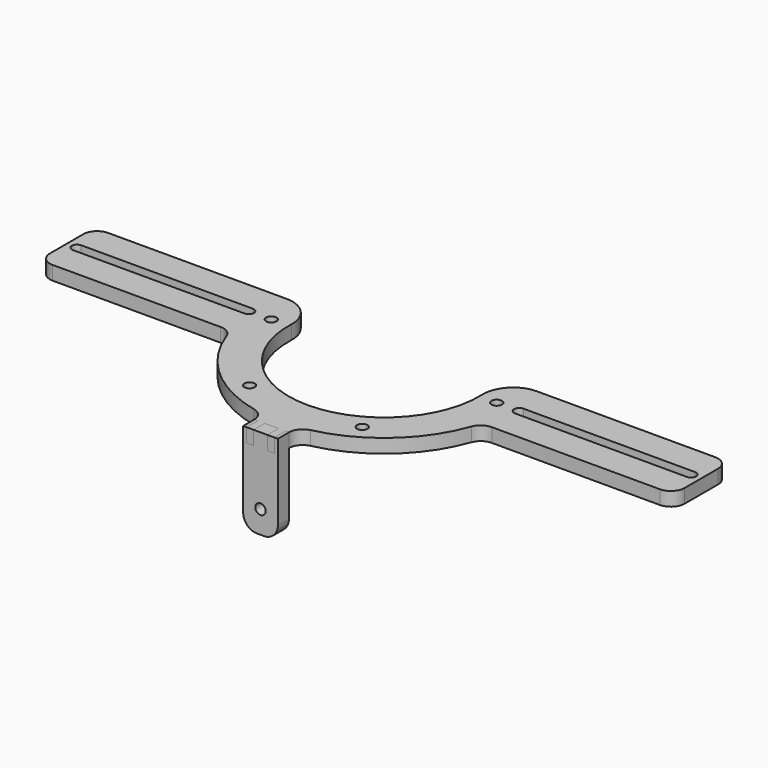
from build123d import *

# Parameters (mm, degrees)
F1_DEPTH      = 4
F3_D          = 3
F5_DEPTH      = 4
F6_W          = 4
F6_H          = 26
F7_DEPTH      = 5
F7_DEPTH_BACK = 5
F8_T1_DEPTH   = 4
F8_T6_DEPTH   = 4
F8_T11_DEPTH  = 4
F8_T13_DEPTH  = 24
F8_2_F1_R     = 4
F8_2_F2_R     = 4
F10_D         = 3
F11_W         = 2
F11_H         = 4
F12_DEPTH     = 4


# Not quite as in the source:
# - a fillet or chamfer that OpenCascade refuses, or shapes differently, is made with other operations: its cross-section is extruded or revolved along the edge and cut away or added
# - a feature names something its author has since deleted; it is built from what else it names


with BuildPart() as f1:
    # F0 (on Top) → F1 (new body)
    with BuildSketch(Plane.XY):
        with BuildLine():
            ThreePointArc((27.4813056295, 1.0138248848), (0, -27.5), (-27.4813056295, 1.0138248848))
            ThreePointArc((-27.4813056295, 1.0138248848), (-29.9018810474, 7.3475680266), (-36.142080737, 10))
            Line((-36.142080737, 10), (-91.5, 10))
            Line((-91.5, 10), (-91.5, -10))
            Line((-91.5, -10), (-36.142080737, -10))
            ThreePointArc((-36.142080737, -10), (-24.6506458841, -28.2594348404), (-5, -37.1651718683))
            Line((-5, -37.1651718683), (-5, -40.5))
            Line((-5, -40.5), (-4, -40.5))
            Line((-4, -40.5), (-4, -44.5))
            Line((-4, -44.5), (-2, -44.5))
            Line((-2, -44.5), (-2, -40.5))
            Line((-2, -40.5), (2, -40.5))
            Line((2, -40.5), (2, -44.5))
            Line((2, -44.5), (4, -44.5))
            Line((4, -44.5), (4, -40.5))
            Line((4, -40.5), (5, -40.5))
            Line((5, -40.5), (5, -37.1651718683))
            ThreePointArc((5, -37.1651718683), (24.6506458841, -28.2594348404), (36.142080737, -10))
            Line((36.142080737, -10), (91.5, -10))
            Line((91.5, -10), (91.5, 10))
            Line((91.5, 10), (36.142080737, 10))
            ThreePointArc((36.142080737, 10), (29.9018810474, 7.3475680266), (27.4813056295, 1.0138248848))
        make_face()
    extrude(amount=F1_DEPTH)

    # F3 (through all)
    with Locations(Plane.XY.offset(4)):
        with Locations((-32.5, 0), (-16.25, -28.145825623), (16.25, -28.145825623), (32.5, 0)):
            Hole(F3_D / 2)

    # F4 (on face) → F5 (cut, through all)
    with BuildSketch(Plane.XY.offset(4)):
        with BuildLine():
            Line((-39, 1.5), (-88.5, 1.5))
            ThreePointArc((-88.5, 1.5), (-90, 0), (-88.5, -1.5))
            Line((-88.5, -1.5), (-39, -1.5))
            ThreePointArc((-39, -1.5), (-37.5, 0), (-39, 1.5))
        make_face()
        with BuildLine():
            Line((39, -1.5), (88.5, -1.5))
            ThreePointArc((88.5, -1.5), (90, 0), (88.5, 1.5))
            Line((88.5, 1.5), (39, 1.5))
            ThreePointArc((39, 1.5), (37.5, 0), (39, -1.5))
        make_face()
    extrude(amount=-F5_DEPTH, mode=Mode.SUBTRACT)

    # F8: fillet of radius 4 on 10 edges, made by hand

    # F8_s2 → F8_t1 (join)
    with BuildSketch(Plane.XY):
        with BuildLine():
            ThreePointArc((-39.0672497112, -10), (-36.7648151694, -10.7290987204), (-35.3017316668, -12.6506024096))
            ThreePointArc((-35.3017316668, -12.6506024096), (-35.7464824281, -11.3330928709), (-36.142080737, -10))
            Line((-36.142080737, -10), (-39.0672497112, -10))
        make_face()
        with BuildLine():
            ThreePointArc((39.0672497112, -10), (36.7648151694, -10.7290987204), (35.3017316668, -12.6506024096))
            ThreePointArc((35.3017316668, -12.6506024096), (35.7464824281, -11.3330928709), (36.142080737, -10))
            Line((36.142080737, -10), (39.0672497112, -10))
        make_face()
    extrude(amount=F8_T1_DEPTH)


with BuildPart() as f7:
    # F6 (on Right) → F7 (new body, two sides)
    with BuildSketch(Plane.YZ) as f7_sk:
        with Locations((-42.5, -9)):
            Rectangle(F6_W, F6_H)
    extrude(amount=F7_DEPTH)
    extrude(f7_sk.sketch, amount=-F7_DEPTH_BACK)

    # F8#2: fillet of radius 4 on 2 edges, made by hand

    # F8_2_f1
    f8_2_f1_edges = [f7.edges().sort_by_distance(p)[0] for p in [
        (-5, -42.5, -22),
    ]]
    fillet(f8_2_f1_edges, radius=F8_2_F1_R)

    # F8_2_f2
    f8_2_f2_edges = [f7.edges().sort_by_distance(p)[0] for p in [
        (5, -42.5, -22),
    ]]
    fillet(f8_2_f2_edges, radius=F8_2_F2_R)

    # F10 (through all)
    with Locations(Plane.XZ.offset(44.5)):
        with Locations((0, -15.5)):
            Hole(F10_D / 2)

    # F11 (on face) → F12 (cut, through all)
    with BuildSketch(Plane.XZ.offset(44.5)):
        with Locations((3, 2)):
            Rectangle(F11_W, F11_H)
        with Locations((-3, 2)):
            Rectangle(F11_W, F11_H)
    extrude(amount=-F12_DEPTH, mode=Mode.SUBTRACT)


with BuildPart() as f8_tool4:
    # F8_s5 → F8_t6 (new body)
    with BuildSketch(Plane.XY):
        with BuildLine():
            ThreePointArc((8.1325301205, -36.6075395764), (5.8799135014, -38.009333562), (5, -40.5123437979))
            Line((5, -40.5123437979), (5, -37.1651718683))
            ThreePointArc((5, -37.1651718683), (6.5721819272, -36.9195940486), (8.1325301205, -36.6075395764))
        make_face()
    extrude(amount=F8_T6_DEPTH)

    split(bisect_by=Plane.XZ.offset(40.5), keep=Keep.BOTTOM)


with BuildPart() as f1_1:
    add(f1.part)

    # F8_t3: union F8_tool4
    add(f8_tool4.part)


with BuildPart() as f8_tool9:
    # F8_s10 → F8_t11 (new body)
    with BuildSketch(Plane.XY):
        with BuildLine():
            ThreePointArc((-8.1325301205, -36.6075395764), (-5.8799135014, -38.009333562), (-5, -40.5123437979))
            Line((-5, -40.5123437979), (-5, -37.1651718683))
            ThreePointArc((-5, -37.1651718683), (-6.5721819272, -36.9195940486), (-8.1325301205, -36.6075395764))
        make_face()
    extrude(amount=F8_T11_DEPTH)

    split(bisect_by=Plane.XZ.offset(40.5), keep=Keep.BOTTOM)


with BuildPart() as f1_2:
    add(f1_1.part)

    # F8_t8: union F8_tool9
    add(f8_tool9.part)

    # F8_s14 → F8_t13 (cut)
    with BuildSketch(Plane.XY.offset(-10)):
        with BuildLine():
            ThreePointArc((91.5, -6), (90.3284271247, -8.8284271247), (87.5, -10))
            Line((87.5, -10), (91.5, -10))
            Line((91.5, -10), (91.5, -6))
        make_face()
        with BuildLine():
            ThreePointArc((-91.5, 6), (-90.3284271247, 8.8284271247), (-87.5, 10))
            Line((-87.5, 10), (-91.5, 10))
            Line((-91.5, 10), (-91.5, 6))
        make_face()
        with BuildLine():
            ThreePointArc((-87.5, -10), (-90.3284271247, -8.8284271247), (-91.5, -6))
            Line((-91.5, -6), (-91.5, -10))
            Line((-91.5, -10), (-87.5, -10))
        make_face()
        with BuildLine():
            ThreePointArc((87.5, 10), (90.3284271247, 8.8284271247), (91.5, 6))
            Line((91.5, 6), (91.5, 10))
            Line((91.5, 10), (87.5, 10))
        make_face()
    extrude(amount=F8_T13_DEPTH, mode=Mode.SUBTRACT)


solid = Compound([f7.part, f1_2.part])
